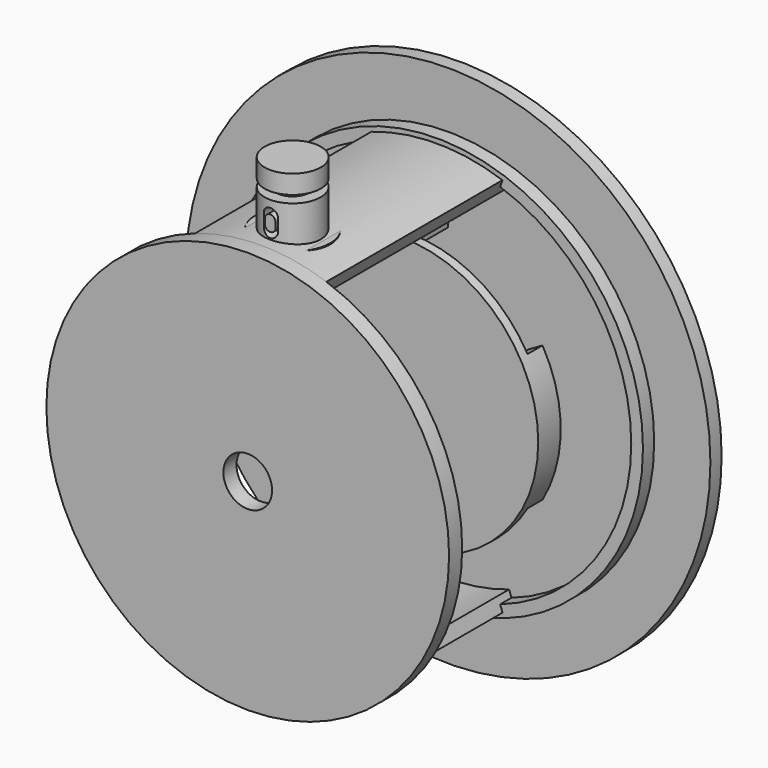
from build123d import *

# Parameters (mm, degrees)
F0_R           = 28
F1_DEPTH       = 1.5
F3_DEPTH       = 5.1
F5_DEPTH       = 25
F6_R           = 21.5
F7_DEPTH       = 1.75
F8_R           = 2.6
F9_DEPTH       = 25
F10_R          = 1.975
F11_DEPTH      = 30
F13_END_RADIUS = 21.5
F12_R          = 3.75
F12_R_2        = 1.875
F13_REACH      = 38.6076017178
F14_W          = 16
F14_H          = 26.820743024
F15_DEPTH      = 25
F15_DEPTH_BACK = 25
F16_R          = 14.5
F17_DEPTH      = 1
F19_DEPTH      = 2
F21_R          = 22.5
F21_R_2        = 20.5
F22_DEPTH      = 1
F23_R          = 22
F23_R_2        = 20.75
F24_DEPTH      = 1.5
F25_R          = 3.1
F26_DEPTH      = 5.5
F28_R          = 3
F28_R_2        = 1.75
F29_DEPTH      = 4
F30_R          = 1.75
F31_DEPTH      = 25
F32_R          = 4
F32_R_2        = 3.1
F33_DEPTH      = 3.5
F36_R          = 3
F37_DEPTH      = 2
F38_R          = 1.25
F39_DEPTH      = 5
F40_R          = 30
F40_R_2        = 29
F41_DEPTH      = 25
F43_DEPTH      = 5
F43_DEPTH_BACK = 5
F45_DEPTH      = 3
F45_DEPTH_BACK = 3


with BuildPart() as f1:
    # F0 (on Front) → F1 (new body)
    with BuildSketch(Plane.XZ):
        Circle(F0_R)
    extrude(amount=F1_DEPTH)

    # F2 (on face) → F3 (join)
    with BuildSketch(Plane.XZ.offset(1.5)):
        with BuildLine():
            ThreePointArc((0, -13), (-13, 0), (0, 13))
            Line((0, 13), (0, 14.5))
            ThreePointArc((0, 14.5), (-14.5, 0), (0, -14.5))
            Line((0, -14.5), (0, -13))
        make_face()
    extrude(amount=F3_DEPTH)

    # F4 (on face) → F5 (join)
    with BuildSketch(Plane.XZ.offset(1.5)):
        with BuildLine():
            Line((6.5113630891, 18.910371512), (6.9997153208, 20.3286493754))
            ThreePointArc((6.9997153208, 20.3286493754), (0, 21.5), (-6.9997153208, 20.3286493754))
            Line((-6.9997153208, 20.3286493754), (-6.5113630891, 18.910371512))
            ThreePointArc((-6.5113630891, 18.910371512), (0, 20), (6.5113630891, 18.910371512))
        make_face()
        with BuildLine():
            ThreePointArc((6.5113630891, -18.910371512), (0, -20), (-6.5113630891, -18.910371512))
            Line((-6.5113630891, -18.910371512), (-6.9997153208, -20.3286493754))
            ThreePointArc((-6.9997153208, -20.3286493754), (0, -21.5), (6.9997153208, -20.3286493754))
            Line((6.9997153208, -20.3286493754), (6.5113630891, -18.910371512))
        make_face()
    extrude(amount=F5_DEPTH)

    # F6 (on face) → F7 (join)
    with BuildSketch(Plane.XZ.offset(26.5)):
        Circle(F6_R)
    extrude(amount=F7_DEPTH)

    # F8 (on face) → F9 (cut)
    with BuildSketch(Plane.XZ.offset(28.25)):
        Circle(F8_R)
    extrude(amount=-F9_DEPTH, mode=Mode.SUBTRACT)

    # F10 (on Top) → F11 (cut)
    with BuildSketch(Plane.XY):
        with Locations((0, -22.25)):
            Circle(F10_R)
    extrude(amount=-F11_DEPTH, mode=Mode.SUBTRACT)

    f13_end = (Plane.ZX.offset(-14) * Cylinder(F13_END_RADIUS, 245.3825308212, mode=Mode.PRIVATE)).faces().sort_by_distance((0, -14, -21.5))[0]
    # F12 (on Top) → F13 (join, up to the whole of a round face its end follows)
    with BuildSketch(Plane.XY):
        with Locations((0, -22.25)):
            Circle(F12_R)
        with Locations((0, -22.25)):
            Circle(F12_R_2, mode=Mode.SUBTRACT)
    f13_long = extrude(amount=-F13_REACH, mode=Mode.PRIVATE)
    add(split(f13_long, bisect_by=f13_end, keep=Keep.BOTTOM, mode=Mode.PRIVATE))

    # F14 (on Right) → F15 (cut, two sides)
    with BuildSketch(Plane.YZ) as f15_sk:
        with Locations((-18.25, 0)):
            Rectangle(F14_W, F14_H)
    extrude(amount=-F15_DEPTH, mode=Mode.SUBTRACT)
    extrude(f15_sk.sketch, amount=F15_DEPTH_BACK, mode=Mode.SUBTRACT)

    # F16 (on face) → F17 (join)
    with BuildSketch(Plane.XZ.offset(6.6)):
        Circle(F16_R)
    extrude(amount=F17_DEPTH)

    # F18 (on face) → F19 (join)
    with BuildSketch(Plane(origin=(0, -6.6, 0), x_dir=(-1, 0, 0), z_dir=(0, 1, 0))):
        with BuildLine():
            Line((-11.0418238983, 6.375), (-12.5573683549, 7.25))
            ThreePointArc((-12.5573683549, 7.25), (-14.5, 0), (-12.5573683549, -7.25))
            Line((-12.5573683549, -7.25), (-11.0418238983, -6.375))
            ThreePointArc((-11.0418238983, -6.375), (-12.75, 0), (-11.0418238983, 6.375))
        make_face()
    extrude(amount=F19_DEPTH)

    # F21 (on face) → F22 (join)
    with BuildSketch(Plane(origin=(0, 0, 0), x_dir=(-1, 0, 0), z_dir=(0, 1, 0))):
        Circle(F21_R)
        Circle(F21_R_2, mode=Mode.SUBTRACT)
    extrude(amount=F22_DEPTH)

    # F23 (on face) → F24 (join)
    with BuildSketch(Plane.XZ.offset(1.5)):
        Circle(F23_R)
        Circle(F23_R_2, mode=Mode.SUBTRACT)
    extrude(amount=F24_DEPTH)

    # F25 (on offset) → F26 (cut)
    with BuildSketch(Plane.XY.offset(15)):
        with Locations((0, -22.25)):
            Circle(F25_R)
    extrude(amount=F26_DEPTH, mode=Mode.SUBTRACT)

    # F28 (on offset) → F29 (join)
    with BuildSketch(Plane.XY.offset(21.25)):
        with Locations((0, -22.25)):
            Circle(F28_R)
        with Locations((0, -22.25)):
            Circle(F28_R_2, mode=Mode.SUBTRACT)
    extrude(amount=F29_DEPTH)

    # F30 (on face) → F31 (cut)
    with BuildSketch(Plane(origin=(0, 0, 20.5), x_dir=(1, 0, 0), z_dir=(0, 0, -1))):
        with Locations((0, 22.25)):
            Circle(F30_R)
    extrude(amount=-F31_DEPTH, mode=Mode.SUBTRACT)

    # F32 (on offset) → F33 (join)
    with BuildSketch(Plane.XY.offset(21.25)):
        with Locations((0, -22.25)):
            Circle(F32_R)
        with Locations((0, -22.25)):
            Circle(F32_R_2, mode=Mode.SUBTRACT)
    extrude(amount=-F33_DEPTH)

    # F40 (on face) → F41 (cut)
    with BuildSketch(Plane.XZ.offset(1.5)):
        Circle(F40_R)
        Circle(F40_R_2, mode=Mode.SUBTRACT)
    extrude(amount=F41_DEPTH, mode=Mode.SUBTRACT)

    # F42 (on offset) → F43 (cut, two sides)
    with BuildSketch(Plane.XZ.offset(22.25)) as f43_sk:
        with BuildLine():
            Line((0.75, 22.4), (0.75, 23.75))
            ThreePointArc((0.75, 23.75), (0, 24.5), (-0.75, 23.75))
            Line((-0.75, 23.75), (-0.75, 22.4))
            ThreePointArc((-0.75, 22.4), (0, 21.65), (0.75, 22.4))
        make_face()
    extrude(amount=-F43_DEPTH, mode=Mode.SUBTRACT)
    extrude(f43_sk.sketch, amount=F43_DEPTH_BACK, mode=Mode.SUBTRACT)


with BuildPart() as f37:
    # F36 (on offset) → F37 (new body)
    with BuildSketch(Plane.XY.offset(28.05)):
        with Locations((0, -22.25)):
            Circle(F36_R)
    extrude(amount=-F37_DEPTH)


with BuildPart() as f39:
    # F38 (on face) → F39 (new body)
    with BuildSketch(Plane(origin=(0, 0, 26.05), x_dir=(1, 0, 0), z_dir=(0, 0, -1))):
        with Locations((0, 22.25)):
            Circle(F38_R)
    extrude(amount=F39_DEPTH)

    # F44 (on offset) → F45 (join, two sides)
    with BuildSketch(Plane.XZ.offset(22.25)) as f45_sk:
        with BuildLine():
            Line((0.575, 22.8), (0.575, 23.3))
            ThreePointArc((0.575, 23.3), (0, 23.875), (-0.575, 23.3))
            Line((-0.575, 23.3), (-0.575, 22.8))
            ThreePointArc((-0.575, 22.8), (0, 22.225), (0.575, 22.8))
        make_face()
    extrude(amount=F45_DEPTH)
    extrude(f45_sk.sketch, amount=-F45_DEPTH_BACK)


solid = Compound([f1.part, f37.part, f39.part])
